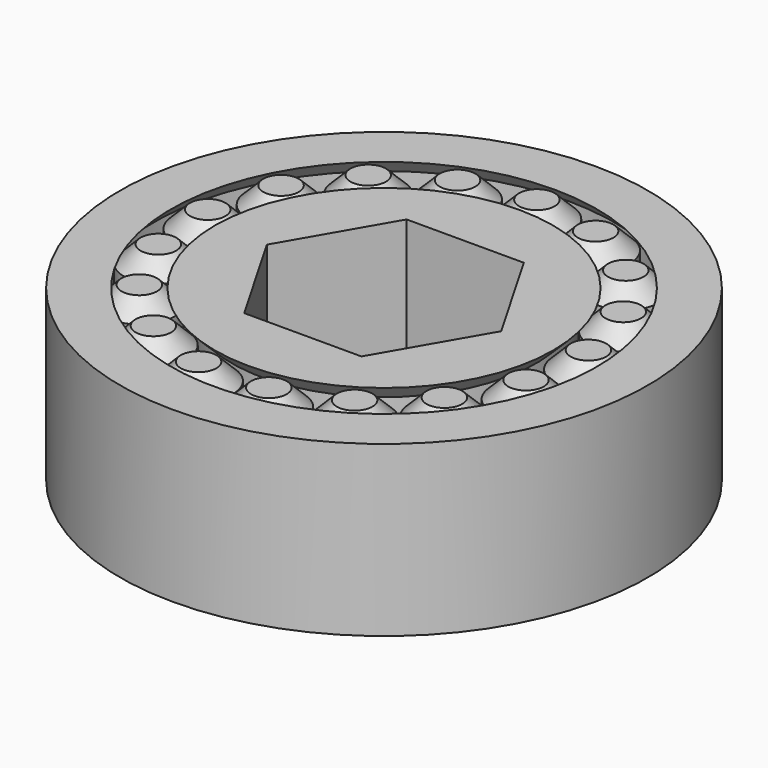
from build123d import *

# Parameters (mm, degrees)
F2_COPIES_COUNT = 17
F5_DEPTH        = 25


# Not quite as in the source:
# - a pattern or mirror of a feature is missing from the dataset's text; its kind, count and spacing are read off the source's solid


with BuildPart() as f1:
    # F0 (on Right) → F1 (revolve)
    with BuildSketch(Plane.YZ):
        Polygon((0, 10), (0, 0), (10, 0), (9, 1), (9, 9), (10, 10), align=None)
    revolve(axis=Axis((0, 0, 5), (0, 0, 1)))

    # F4 (on face) → F5 (cut)
    with BuildSketch(Plane.XY.offset(10)):
        Polygon((3.4641016151, 6), (-3.4641016151, 6), (-6.9282032303, 0), (-3.4641016151, -6), (3.4641016151, -6), (6.9282032303, 0), align=None)
    extrude(amount=-F5_DEPTH, mode=Mode.SUBTRACT)


with BuildPart() as f2:
    # F0 (on Right) → F2 (revolve)
    with BuildSketch(Plane.YZ):
        Polygon((9.25, 9), (9.25, 1), (10.25, 0), (11.3, 0), (11.3, 10), (10.25, 10), align=None)
    revolve(axis=Axis((0, 11.3, 5), (0, 0, 1)))


with BuildPart() as f2_copies_1:
    # F2_copies: instance of F2
    add(f2.part.rotate(Axis((0, 0, 0), (0, 0, 1)), 1 * 360 / F2_COPIES_COUNT))


with BuildPart() as f2_copies_2:
    # F2_copies: instance of F2
    add(f2.part.rotate(Axis((0, 0, 0), (0, 0, 1)), 2 * 360 / F2_COPIES_COUNT))


with BuildPart() as f2_copies_3:
    # F2_copies: instance of F2
    add(f2.part.rotate(Axis((0, 0, 0), (0, 0, 1)), 3 * 360 / F2_COPIES_COUNT))


with BuildPart() as f2_copies_4:
    # F2_copies: instance of F2
    add(f2.part.rotate(Axis((0, 0, 0), (0, 0, 1)), 4 * 360 / F2_COPIES_COUNT))


with BuildPart() as f2_copies_5:
    # F2_copies: instance of F2
    add(f2.part.rotate(Axis((0, 0, 0), (0, 0, 1)), 5 * 360 / F2_COPIES_COUNT))


with BuildPart() as f2_copies_6:
    # F2_copies: instance of F2
    add(f2.part.rotate(Axis((0, 0, 0), (0, 0, 1)), 6 * 360 / F2_COPIES_COUNT))


with BuildPart() as f2_copies_7:
    # F2_copies: instance of F2
    add(f2.part.rotate(Axis((0, 0, 0), (0, 0, 1)), 7 * 360 / F2_COPIES_COUNT))


with BuildPart() as f2_copies_8:
    # F2_copies: instance of F2
    add(f2.part.rotate(Axis((0, 0, 0), (0, 0, 1)), 8 * 360 / F2_COPIES_COUNT))


with BuildPart() as f2_copies_9:
    # F2_copies: instance of F2
    add(f2.part.rotate(Axis((0, 0, 0), (0, 0, 1)), 9 * 360 / F2_COPIES_COUNT))


with BuildPart() as f2_copies_10:
    # F2_copies: instance of F2
    add(f2.part.rotate(Axis((0, 0, 0), (0, 0, 1)), 10 * 360 / F2_COPIES_COUNT))


with BuildPart() as f2_copies_11:
    # F2_copies: instance of F2
    add(f2.part.rotate(Axis((0, 0, 0), (0, 0, 1)), 11 * 360 / F2_COPIES_COUNT))


with BuildPart() as f2_copies_12:
    # F2_copies: instance of F2
    add(f2.part.rotate(Axis((0, 0, 0), (0, 0, 1)), 12 * 360 / F2_COPIES_COUNT))


with BuildPart() as f2_copies_13:
    # F2_copies: instance of F2
    add(f2.part.rotate(Axis((0, 0, 0), (0, 0, 1)), 13 * 360 / F2_COPIES_COUNT))


with BuildPart() as f2_copies_14:
    # F2_copies: instance of F2
    add(f2.part.rotate(Axis((0, 0, 0), (0, 0, 1)), 14 * 360 / F2_COPIES_COUNT))


with BuildPart() as f2_copies_15:
    # F2_copies: instance of F2
    add(f2.part.rotate(Axis((0, 0, 0), (0, 0, 1)), 15 * 360 / F2_COPIES_COUNT))


with BuildPart() as f2_copies_16:
    # F2_copies: instance of F2
    add(f2.part.rotate(Axis((0, 0, 0), (0, 0, 1)), 16 * 360 / F2_COPIES_COUNT))


with BuildPart() as f3:
    # F0 (on Right) → F3 (revolve)
    with BuildSketch(Plane.YZ):
        Polygon((15.6, 10), (12.6, 10), (13.6, 9), (13.6, 1), (12.6, 0), (15.6, 0), align=None)
    revolve(axis=Axis((0, 0, 5), (0, 0, 1)))


solid = Compound([f1.part, f2.part, f2_copies_1.part, f2_copies_2.part, f2_copies_3.part, f2_copies_4.part, f2_copies_5.part, f2_copies_6.part, f2_copies_7.part, f2_copies_8.part, f2_copies_9.part, f2_copies_10.part, f2_copies_11.part, f2_copies_12.part, f2_copies_13.part, f2_copies_14.part, f2_copies_15.part, f2_copies_16.part, f3.part])
